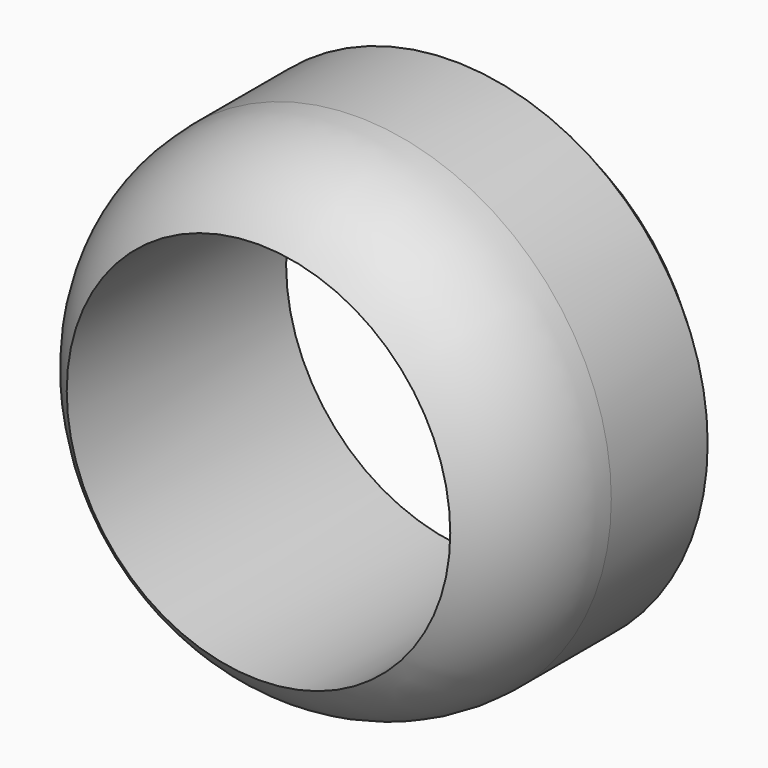
from build123d import *

# Parameters (mm, degrees)
F0_R     = 41.7073575722
F0_R_2   = 31.46793235
F1_DEPTH = 45
F3_SIZE  = 5


# Not quite as in the source:
# - a fillet or chamfer that OpenCascade refuses, or shapes differently, is made with other operations: its cross-section is extruded or revolved along the edge and cut away or added


with BuildPart() as f1:
    # F0 (on Front) → F1 (new body)
    with BuildSketch(Plane.XZ):
        Circle(F0_R)
        Circle(F0_R_2, mode=Mode.SUBTRACT)
    extrude(amount=F1_DEPTH)

    # F2: fillet of radius 25.1078210487 on 1 edges, made by hand

    # F2_s1 → F2_t2 (revolve, cut)
    with BuildSketch(Plane.XY):
        with BuildLine():
            ThreePointArc((41.7073575722, -24.7680084183), (39.0017205633, -36.1057695757), (31.46793235, -45))
            Line((31.46793235, -45), (41.7073575722, -45))
            Line((41.7073575722, -45), (41.7073575722, -24.7680084183))
        make_face()
    revolve(axis=Axis((0, -45, 0), (0, -1, 0)), mode=Mode.SUBTRACT)

    # F3
    f3_edges = [f1.edges().sort_by_distance(p)[0] for p in [
        (-41.707358, 0, 0),
    ]]
    chamfer(f3_edges, length=F3_SIZE)


solid = f1.part
